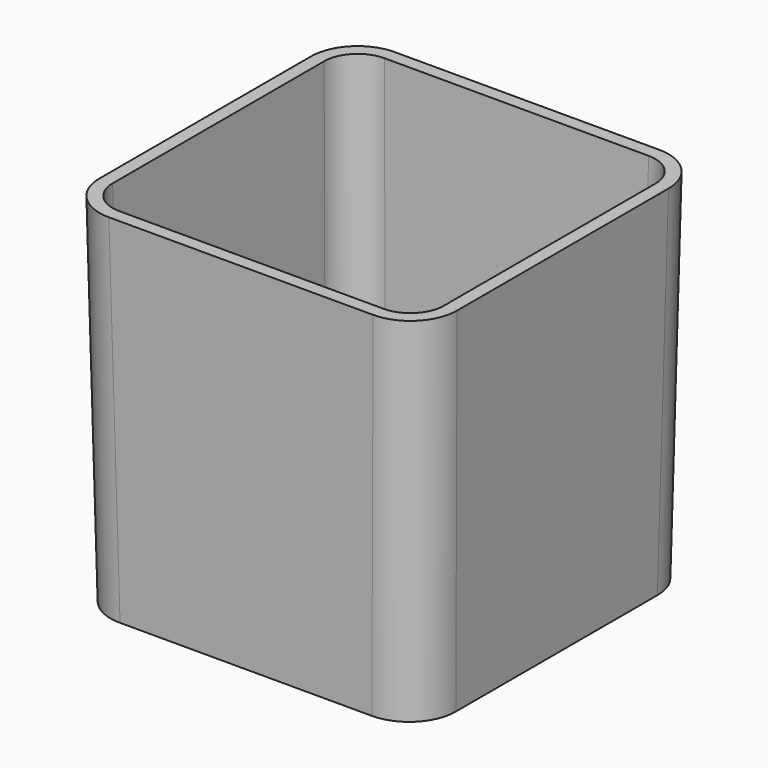
from build123d import *

# Parameters (mm, degrees)
F0_W                   = 69
F0_H                   = 69
F1_DEPTH               = 69
DRAFT_F1_DRAFTED_ANGLE = 1
F2_R                   = 9
F3_T                   = -2.54


# Not quite as in the source:
# - an extrude with a draft is written as a straight extrude whose walls are then drafted


with BuildPart() as f1:
    # F0 (on Top) → F1 (new body)
    with BuildSketch(Plane.XY):
        Rectangle(F0_W, F0_H)
    extrude(amount=-F1_DEPTH)

    # draft_F1_drafted
    draft_f1_drafted_walls = [f1.faces().sort_by_distance(p)[0] for p in [
        (34.5, 0, -46),
        (0, 34.5, -46),
        (-34.5, 0, -46),
        (0, -34.5, -46),
    ]]
    draft(draft_f1_drafted_walls, neutral_plane=Plane(origin=(0, 0, 0), x_dir=(1, 0, 0), z_dir=(0, 0, -1)), angle=DRAFT_F1_DRAFTED_ANGLE)

    # F2
    f2_edges = [f1.edges().sort_by_distance(p)[0] for p in [
        (33.8978, -33.8978, -34.5),
        (33.8978, 33.8978, -34.5),
        (-33.8978, 33.8978, -34.5),
        (-33.8978, -33.8978, -34.5),
    ]]
    fillet(f2_edges, radius=F2_R)

    # F3
    f3_openings = [f1.faces().sort_by_distance(p)[0] for p in [
        (0, 0, 0),
    ]]
    offset(amount=F3_T, openings=f3_openings)


solid = f1.part
